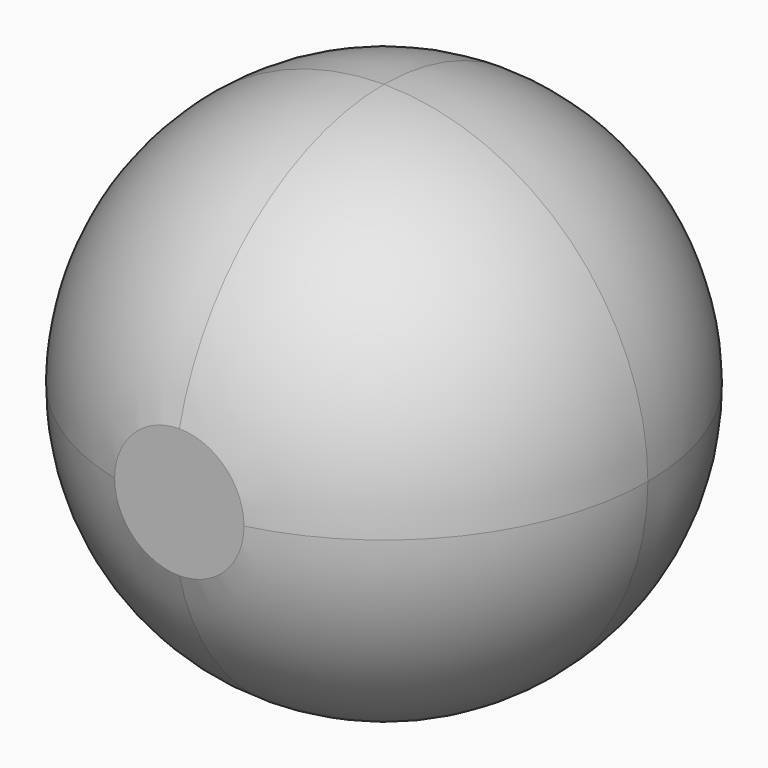
from build123d import *

# Parameters (mm, degrees)
F0_W     = 30
F0_H     = 30
F1_DEPTH = 30
F2_R     = 14.99999
F3_W     = 1.993669197
F3_H     = 26.7333146185
F4_DEPTH = 30.001


# Not quite as in the source:
# - a fillet or chamfer is up to 0.001 mm smaller than in the source, because OpenCascade refuses the exact size


with BuildPart() as f1:
    # F0 (on Front) → F1 (new body)
    with BuildSketch(Plane.XZ):
        with Locations((-15, 15)):
            Rectangle(F0_W, F0_H)
    extrude(amount=F1_DEPTH)

    # F2 (radius 15 in the source; OpenCascade refuses exactly that, so slightly less here)
    f2_edges = [f1.edges().sort_by_distance(p)[0] for p in [
        (-15, -30, 0),
        (0, -30, 15),
        (-15, -30, 30),
        (-30, -30, 15),
        (0, -15, 30),
        (-30, -15, 30),
        (-15, 0, 30),
        (0, -15, 0),
        (0, 0, 15),
        (-15, 0, 0),
        (-30, 0, 15),
        (-30, -15, 0),
    ]]
    fillet(f2_edges, radius=F2_R)

    # F3 (on Right) → F4 (cut, through all)
    with BuildSketch(Plane.YZ):
        with Locations((-30.5394129828, 13.3666573092)):
            Rectangle(F3_W, F3_H)
    extrude(amount=-F4_DEPTH, mode=Mode.SUBTRACT)


solid = f1.part
